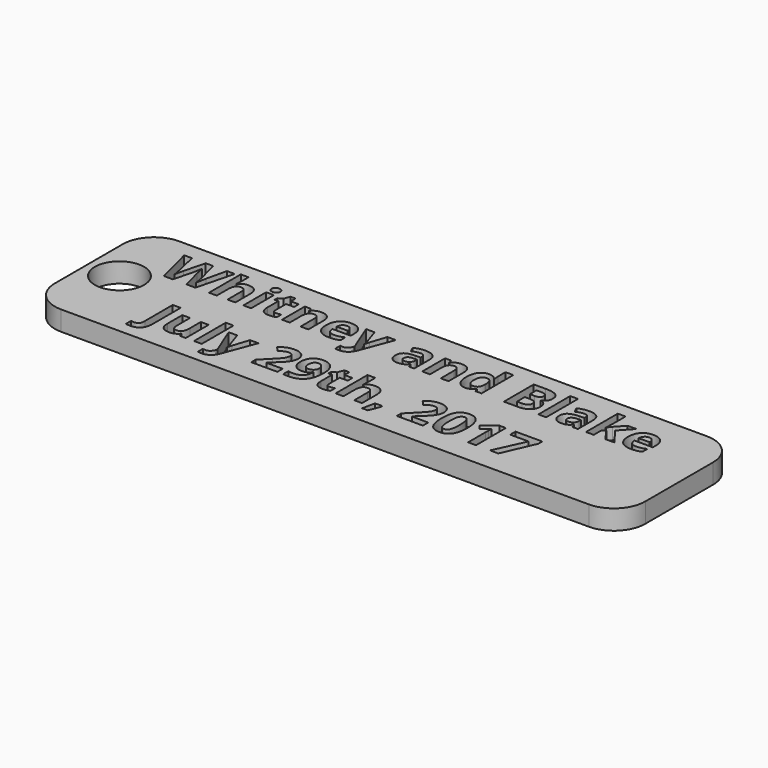
from build123d import *

# Parameters (mm, degrees)
F0_W         = 38.1
F0_H         = 9.525
F1_DEPTH     = 1.27
F2_TEXT_SIZE = 3.3748546753
F3_DEPTH     = 0.762
F4_R         = 1.5875
F5_DEPTH     = 1.27
F6_R         = 2.023593808


# Not quite as in the source:
# - Text() gives the source's letters only with a copy of the font that has no kerning and outlines rounded to 1/6400 em; it was checked with that copy


with BuildPart() as f1:
    # F0 (on Top) → F1 (new body)
    with BuildSketch(Plane.XY):
        with Locations((19.05, -4.7625)):
            Rectangle(F0_W, F0_H)
    extrude(amount=F1_DEPTH)

    # F2 (on face) → F3 (cut)
    with BuildSketch(Plane.XY.offset(1.27)):
        with Locations((3.175, -3.4458953662)):
            Text('Whitney and Blake', F2_TEXT_SIZE, font='Open Sans', font_style=FontStyle.BOLD, text_align=(TextAlign.LEFT, TextAlign.BOTTOM))
        with Locations((5.8058046836, -8.0356977246)):
            Text('July 29th, 2017', F2_TEXT_SIZE, font='Open Sans', font_style=FontStyle.BOLD, text_align=(TextAlign.LEFT, TextAlign.BOTTOM))
    extrude(amount=-F3_DEPTH, mode=Mode.SUBTRACT)

    # F4 (on face) → F5 (cut, through all)
    with BuildSketch(Plane.XY.offset(1.27)):
        with Locations((2.032, -4.826)):
            Circle(F4_R)
    extrude(amount=-F5_DEPTH, mode=Mode.SUBTRACT)

    # F6
    f6_edges = [f1.edges().sort_by_distance(p)[0] for p in [
        (38.1, -9.525, 0.635),
        (38.1, 0, 0.635),
        (0, 0, 0.635),
        (0, -9.525, 0.635),
    ]]
    fillet(f6_edges, radius=F6_R)


solid = f1.part
